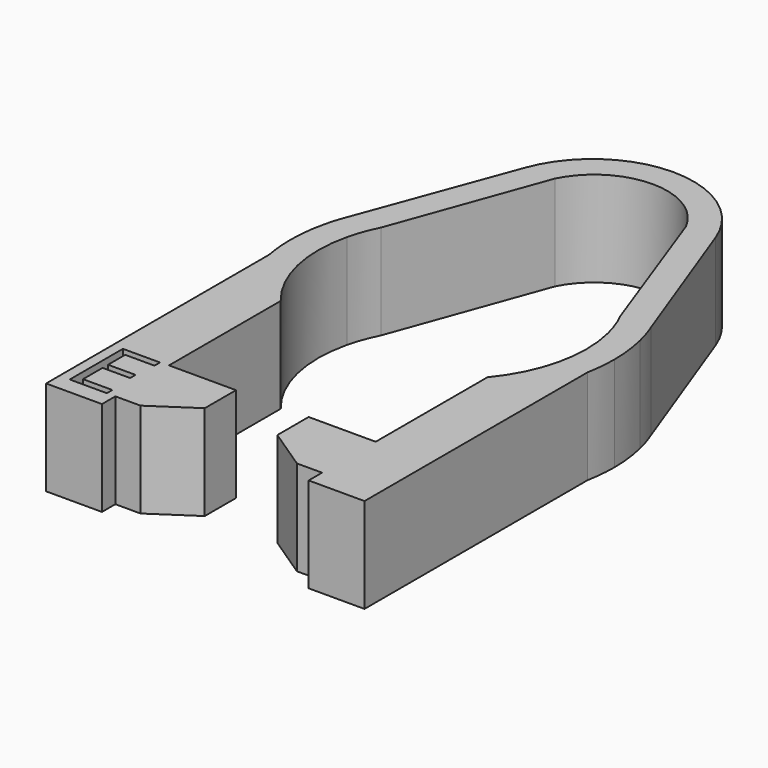
from build123d import *

# Parameters (mm, degrees)
F0_TEXT_SIZE = 8.3333333333
F1_DEPTH     = 8.5
F2_DEPTH     = 1


# Not quite as in the source:
# - Text() gives the source's letters only with a copy of the font that has no kerning and outlines rounded to 1/6400 em; it was checked with that copy


with BuildPart() as f1:
    # F0 (on Top) → F1 (new body)
    with BuildSketch(Plane.XY):
        with BuildLine():
            ThreePointArc((-9.25, -7.6444424257), (-11.6891485981, -2.7136331829), (-11.6717637121, 2.7874597484))
            ThreePointArc((-11.6717637121, 2.7874597484), (-11.2656904289, 4.1333060811), (-10.7050113586, 5.42242859))
            Line((-10.7050113586, 5.42242859), (-5.8459149373, 18.8072078091))
            ThreePointArc((-5.8459149373, 18.8072078091), (0, 22.4041745059), (5.8459149373, 18.8072078091))
            Line((5.8459149373, 18.8072078091), (10.7050113586, 5.42242859))
            ThreePointArc((10.7050113586, 5.42242859), (11.2656904289, 4.1333060811), (11.6717637121, 2.7874597484))
            ThreePointArc((11.6717637121, 2.7874597484), (11.6891485981, -2.7136331829), (9.25, -7.6444424257))
            Line((9.25, -7.6444424257), (9.25, -11.1663557171))
            Line((9.25, -11.1663557171), (9.25, -20.1444424257))
            Line((9.25, -20.1444424257), (3.25, -20.1444424257))
            Line((3.25, -20.1444424257), (3.25, -21.1444424257))
            Line((3.25, -21.1444424257), (3.25, -23.6444424257))
            Line((3.25, -23.6444424257), (7, -26.1444424257))
            Line((7, -26.1444424257), (9.25, -26.1444424257))
            Line((9.25, -26.1444424257), (9.25, -27.6444424257))
            Line((9.25, -27.6444424257), (14.25, -27.6444424257))
            Line((14.25, -27.6444424257), (14.25, -21.4303609628))
            Line((14.25, -21.4303609628), (14.25, -2.6809513237))
            ThreePointArc((14.25, -2.6809513237), (14.437364718, -1.3462912018), (14.5, 0))
            ThreePointArc((14.5, 0), (14.400503927, 1.6957259941), (14.1033811521, 3.3681805293))
            ThreePointArc((14.1033811521, 3.3681805293), (13.8091695526, 4.4223111907), (13.4362898945, 5.4512488358))
            Line((13.4362898945, 5.4512488358), (8.4985279846, 18.8072078091))
            ThreePointArc((8.4985279846, 18.8072078091), (0, 24.7259901099), (-8.4985279846, 18.8072078091))
            Line((-8.4985279846, 18.8072078091), (-13.4362898945, 5.4512488358))
            ThreePointArc((-13.4362898945, 5.4512488358), (-13.8091695526, 4.4223111907), (-14.1033811521, 3.3681805293))
            ThreePointArc((-14.1033811521, 3.3681805293), (-14.400503927, 1.6957259941), (-14.5, 0))
            ThreePointArc((-14.5, 0), (-14.437364718, -1.3462912018), (-14.25, -2.6809513237))
            Line((-14.25, -2.6809513237), (-14.25, -21.1444424257))
            Line((-14.25, -21.1444424257), (-14.25, -27.6444424257))
            Line((-14.25, -27.6444424257), (-9.25, -27.6444424257))
            Line((-9.25, -27.6444424257), (-9.25, -26.1444424257))
            Line((-9.25, -26.1444424257), (-7, -26.1444424257))
            Line((-7, -26.1444424257), (-3.25, -23.6444424257))
            Line((-3.25, -23.6444424257), (-3.25, -21.1444424257))
            Line((-3.25, -21.1444424257), (-3.25, -20.1444424257))
            Line((-3.25, -20.1444424257), (-9.25, -20.1444424257))
            Line((-9.25, -20.1444424257), (-9.25, -11.1663557171))
            Line((-9.25, -11.1663557171), (-9.25, -7.6444424257))
        make_face()
        Polygon((-10.0158854167, -25.5259528424), (-10.0158854167, -26.1444424257), (-13.3322916667, -26.1444424257), (-13.3322916667, -20.1952236757), (-10.0158854167, -20.1952236757), (-10.0158854167, -20.809807009), (-12.6408854167, -20.809807009), (-12.6408854167, -22.7264736757), (-10.1747395833, -22.7264736757), (-10.1747395833, -23.337150759), (-12.6408854167, -23.337150759), (-12.6408854167, -25.5259528424), align=None, mode=Mode.SUBTRACT)
        with Locations((-14.15, -26.1444424257)):
            Text('E', F0_TEXT_SIZE, font='Open Sans', text_align=(TextAlign.LEFT, TextAlign.BOTTOM))
    extrude(amount=-F1_DEPTH)

    # F0 (on Top) → F2 (cut)
    with BuildSketch(Plane.XY):
        with Locations((-14.15, -26.1444424257)):
            Text('E', F0_TEXT_SIZE, font='Open Sans', text_align=(TextAlign.LEFT, TextAlign.BOTTOM))
    extrude(amount=-F2_DEPTH, mode=Mode.SUBTRACT)


solid = f1.part
